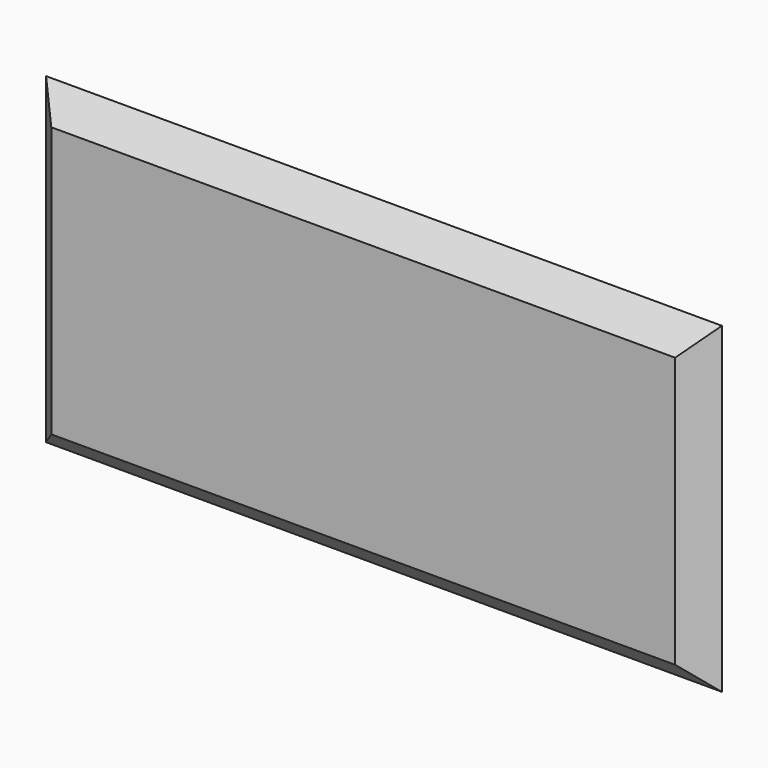
from build123d import *

# Parameters (mm, degrees)
F0_W     = 165.1000007248
F0_H     = 78.7400007248
F1_DEPTH = 6.35
F2_SIZE  = 6.34999


# Not quite as in the source:
# - a fillet or chamfer is up to 0.001 mm smaller than in the source, because OpenCascade refuses the exact size


with BuildPart() as f1:
    # F0 (on Front) → F1 (new body)
    with BuildSketch(Plane.XZ):
        Rectangle(F0_W, F0_H)
    extrude(amount=F1_DEPTH)

    # F2 (size 6.35 in the source; OpenCascade refuses exactly that, so slightly less here)
    f2_edges = [f1.edges().sort_by_distance(p)[0] for p in [
        (0, -6.35, -39.37),
        (82.55, -6.35, 0),
        (0, -6.35, 39.37),
        (-82.55, -6.35, 0),
    ]]
    chamfer(f2_edges, length=F2_SIZE)


solid = f1.part
